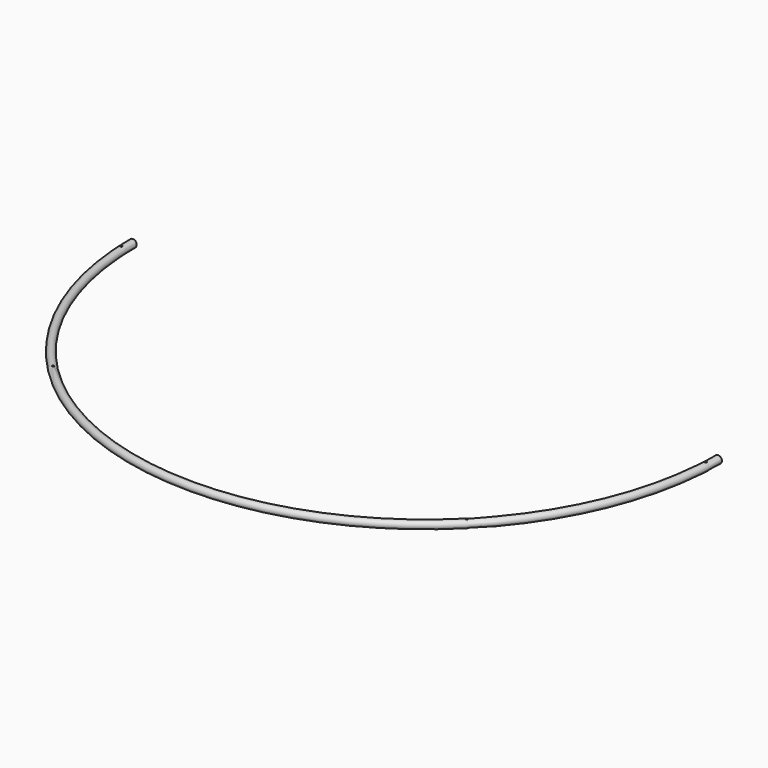
from build123d import *
from build123d import SkipClean  # not in build123d's __all__

# Parameters (mm, degrees)
F0_R          = 19.05
F0_R_2        = 15.85
F1_ANGLE      = 180
F2_R          = 5.25
F3_DEPTH      = 19.0510001
F3_DEPTH_BACK = 19.0510001
F4_R          = 5
F5_DEPTH      = 19.0510001013
F5_DEPTH_BACK = 19.0510001008


with BuildPart() as f1:
    # F0 (on Front) → F1 (revolve)
    with BuildSketch(Plane.XZ):
        with Locations((-1450, 0)):
            Circle(F0_R)
        with Locations((-1450, 0)):
            Circle(F0_R_2, mode=Mode.SUBTRACT)
    revolve(axis=Axis((0, 0, 190.0846064091), (0, 0, 1)), revolution_arc=F1_ANGLE)

    # F2 (on Top) → F3 (cut, two sides)
    with BuildSketch(Plane.XY) as f3_sk:
        with Locations((-1448.0590457575, -75)):
            Circle(F2_R)
        with Locations((1448.0590457575, -75)):
            Circle(F2_R)
    with SkipClean():  # cleaning this boolean's faces spoils the solid; the shape is the same uncleaned
        extrude(amount=-F3_DEPTH, mode=Mode.SUBTRACT)
        extrude(f3_sk.sketch, amount=F3_DEPTH_BACK, mode=Mode.SUBTRACT)

    # F4 (on Top) → F5 (cut, two sides)
    with BuildSketch(Plane.XY) as f5_sk:
        with Locations((-1025.3048327205, -1025.3048327205)):
            Circle(F4_R)
        with Locations((1025.3048327205, -1025.3048327205)):
            Circle(F4_R)
    with SkipClean():  # cleaning this boolean's faces spoils the solid; the shape is the same uncleaned
        extrude(amount=-F5_DEPTH, mode=Mode.SUBTRACT)
        extrude(f5_sk.sketch, amount=F5_DEPTH_BACK, mode=Mode.SUBTRACT)


solid = f1.part
